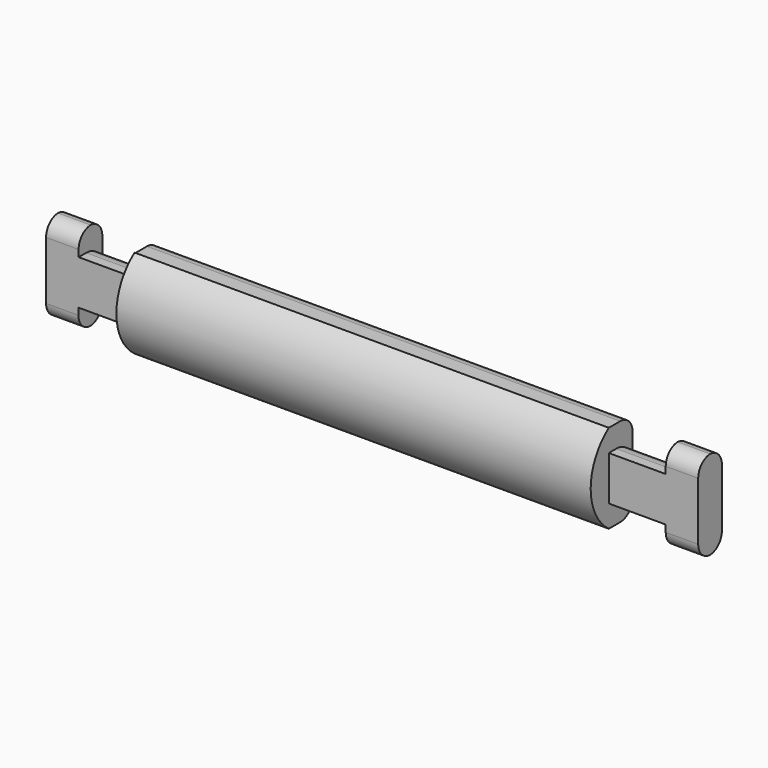
from build123d import *

# Parameters (mm, degrees)
F1_DEPTH    = 6.35
F2_T1_DEPTH = 23.4696
F2_T3_DEPTH = 117.8964839186
F2_T5_DEPTH = 23.4799160814
F2_T7_DEPTH = 117.9413513149
F2_T9_DEPTH = 23.4350486851
F3_R        = 4.318
F5_DEPTH    = 101.6


# Not quite as in the source:
# - a fillet or chamfer that OpenCascade refuses, or shapes differently, is made with other operations: its cross-section is extruded or revolved along the edge and cut away or added


with BuildPart() as f1:
    # F0 (on Front) → F1 (new body)
    with BuildSketch(Plane.XZ):
        Polygon((69.85, -9.525), (69.85, 9.525), (62.8904, 9.525), (62.8904, 4.7625), (50.6984, 4.7625), (50.6984, 9.525), (-50.6880839186, 9.525), (-50.6880839186, 4.7625), (-62.8800839186, 4.7625), (-62.8800839186, 9.525), (-69.85, 9.525), (-69.85, -9.525), (-62.9249513149, -9.525), (-62.9249513149, -4.7625), (-50.7329513149, -4.7625), (-50.7329513149, -9.525), (50.6984, -9.525), (50.6984, -4.7625), (62.8904, -4.7625), (62.8904, -9.525), align=None)
    extrude(amount=F1_DEPTH)

    # F2: fillet of radius 3.302 on 10 edges, made by hand

    # F2_s2 → F2_t1 (cut)
    with BuildSketch(Plane.YZ.offset(54.6354)):
        with BuildLine():
            ThreePointArc((-3.302, 9.525), (-0.9671334085, 8.5578665915), (0, 6.223))
            Line((0, 6.223), (0, 9.525))
            Line((0, 9.525), (-3.302, 9.525))
        make_face()
        with BuildLine():
            ThreePointArc((-3.048, 9.525), (-5.3828665915, 8.5578665915), (-6.35, 6.223))
            Line((-6.35, 6.223), (-6.35, 9.525))
            Line((-6.35, 9.525), (-3.048, 9.525))
        make_face()
        with BuildLine():
            ThreePointArc((-3.302, -9.525), (-0.9671334085, -8.5578665915), (0, -6.223))
            Line((0, -6.223), (0, -9.525))
            Line((0, -9.525), (-3.302, -9.525))
        make_face()
        with BuildLine():
            ThreePointArc((-3.048, -9.525), (-5.3828665915, -8.5578665915), (-6.35, -6.223))
            Line((-6.35, -6.223), (-6.35, -9.525))
            Line((-6.35, -9.525), (-3.048, -9.525))
        make_face()
    extrude(amount=F2_T1_DEPTH, mode=Mode.SUBTRACT)

    # F2_s4 → F2_t3 (cut)
    with BuildSketch(Plane.YZ.offset(-58.9430839186)):
        with BuildLine():
            ThreePointArc((-3.302, 9.525), (-0.9671334085, 8.5578665915), (0, 6.223))
            Line((0, 6.223), (0, 9.525))
            Line((0, 9.525), (-3.302, 9.525))
        make_face()
    extrude(amount=F2_T3_DEPTH, mode=Mode.SUBTRACT)

    # F2_s6 → F2_t5 (cut)
    with BuildSketch(Plane.YZ.offset(-78.105)):
        with BuildLine():
            ThreePointArc((-3.302, 9.525), (-0.9671334085, 8.5578665915), (0, 6.223))
            Line((0, 6.223), (0, 9.525))
            Line((0, 9.525), (-3.302, 9.525))
        make_face()
        with BuildLine():
            ThreePointArc((-3.048, 9.525), (-5.3828665915, 8.5578665915), (-6.35, 6.223))
            Line((-6.35, 6.223), (-6.35, 9.525))
            Line((-6.35, 9.525), (-3.048, 9.525))
        make_face()
    extrude(amount=F2_T5_DEPTH, mode=Mode.SUBTRACT)

    # F2_s8 → F2_t7 (cut)
    with BuildSketch(Plane.YZ.offset(-58.9879513149)):
        with BuildLine():
            ThreePointArc((-3.302, -9.525), (-0.9671334085, -8.5578665915), (0, -6.223))
            Line((0, -6.223), (0, -9.525))
            Line((0, -9.525), (-3.302, -9.525))
        make_face()
    extrude(amount=F2_T7_DEPTH, mode=Mode.SUBTRACT)

    # F2_s10 → F2_t9 (cut)
    with BuildSketch(Plane.YZ.offset(-78.105)):
        with BuildLine():
            ThreePointArc((-3.302, -9.525), (-0.9671334085, -8.5578665915), (0, -6.223))
            Line((0, -6.223), (0, -9.525))
            Line((0, -9.525), (-3.302, -9.525))
        make_face()
        with BuildLine():
            ThreePointArc((-3.048, -9.525), (-5.3828665915, -8.5578665915), (-6.35, -6.223))
            Line((-6.35, -6.223), (-6.35, -9.525))
            Line((-6.35, -9.525), (-3.048, -9.525))
        make_face()
    extrude(amount=F2_T9_DEPTH, mode=Mode.SUBTRACT)

    # F3
    f3_edges = [f1.edges().sort_by_distance(p)[0] for p in [
        (-56.784084, 0, 4.7625),
        (-56.828951, 0, -4.7625),
        (56.7944, 0, -4.7625),
        (56.7944, 0, 4.7625),
    ]]
    fillet(f3_edges, radius=F3_R)

    # F4 (on face) → F5 (join)
    with BuildSketch(Plane.YZ.offset(50.6984)):
        with BuildLine():
            Line((-6.35, 4.7625), (-6.35, 9.525))
            ThreePointArc((-6.35, 9.525), (-11.2043924939, 0.0067562208), (-6.35, -9.5114875585))
            Line((-6.35, -9.5114875585), (-6.35, -4.8156534322))
            Line((-6.35, -4.8156534322), (-6.35, 4.7625))
        make_face()
    extrude(amount=-F5_DEPTH)


solid = f1.part
